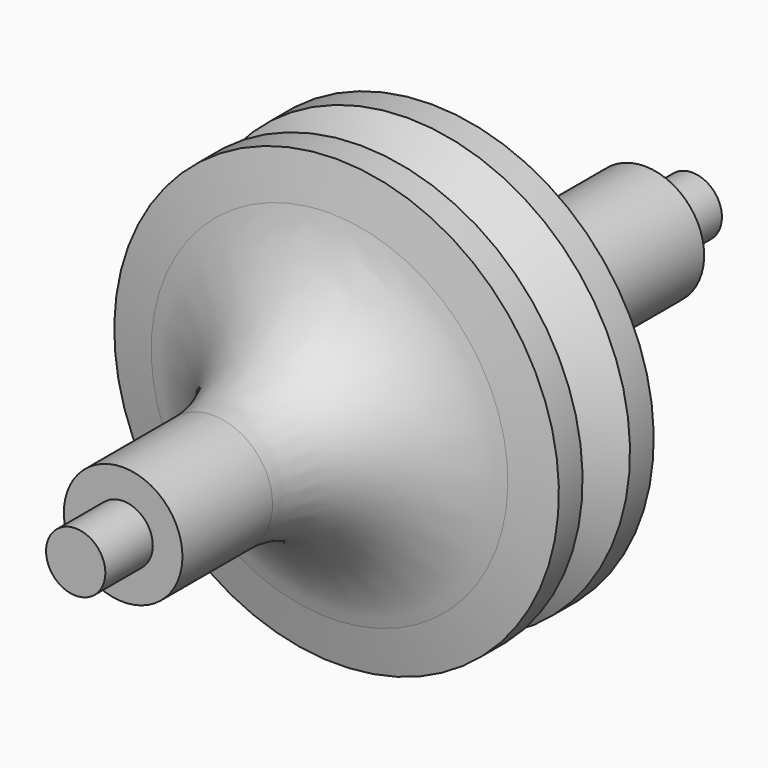
from build123d import *

# Parameters (mm, degrees)
F2_R = 5
F3_R = 5


with BuildPart() as f1:
    # F0 (on Right) → F1 (revolve)
    with BuildSketch(Plane.YZ):
        Polygon((-39.0091740638, 9.247707203), (-26.0091740638, 9.247707203), (-13.0091740638, 9.247707203), (-13.0091740638, 10.247707203), (-15.0091740638, 10.247707203), (-15.0091740638, 11.247707203), (-22.9062791914, 11.247707203), (-24.0091740638, 16.747707203), (-25.0091740638, 16.747707203), (-26.0091740638, 15.4484901577), (-27.0091740638, 16.747707203), (-28.0091740638, 16.747707203), (-29.1120689362, 11.247707203), (-37.0091740638, 11.247707203), (-37.0091740638, 10.247707203), (-39.0091740638, 10.247707203), align=None)
    revolve(axis=Axis((0, -19.5091740638, 9.247707203), (0, 1, 0)))

    # F2
    f2_edges = [f1.edges().sort_by_distance(p)[0] for p in [
        (0, -29.112069, 7.247707),
    ]]
    fillet(f2_edges, radius=F2_R)

    # F3
    f3_edges = [f1.edges().sort_by_distance(p)[0] for p in [
        (0, -22.906279, 7.247707),
    ]]
    fillet(f3_edges, radius=F3_R)


solid = f1.part
